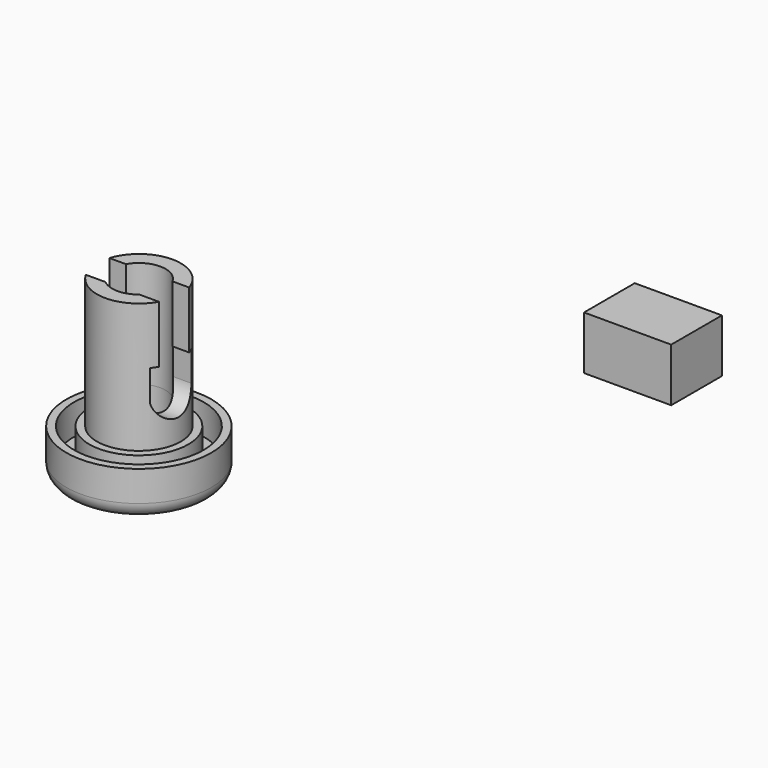
from build123d import *

# Parameters (mm, degrees)
F1_W      = 11.4284157753
F1_H      = 8.3115845919
F2_DEPTH  = 7
F4_R      = 9.5
F4_R_2    = 6.5
F4_R_3    = 5.5
F5_DEPTH  = 2
F0_R      = 5.5
F0_R_2    = 3.5
F6_DEPTH  = 7
F7_DEPTH  = 14
F8_DEPTH  = 12.5
F9_R      = 1.99999
F10_R     = 9.5
F10_R_2   = 8.5
F11_DEPTH = 4
F12_DEPTH = 4


# Not quite as in the source:
# - a fillet or chamfer is up to 0.001 mm smaller than in the source, because OpenCascade refuses the exact size


with BuildPart() as f2:
    # F1 (on Top) → F2 (new body)
    with BuildSketch(Plane.XY):
        with Locations((29.1647613049, 47.7915927768)):
            Rectangle(F1_W, F1_H)
    extrude(amount=-F2_DEPTH)


with BuildPart() as f5:
    # F4 (on face) → F5 (new body)
    with BuildSketch(Plane(origin=(0, 0, -7), x_dir=(1, 0, 0), z_dir=(0, 0, -1))):
        Circle(F4_R)
        Circle(F4_R_2, mode=Mode.SUBTRACT)
        Circle(F4_R_2)
        Circle(F4_R_3, mode=Mode.SUBTRACT)
        Circle(F4_R_3)
    extrude(amount=F5_DEPTH)

    # F0 (on Top) → F6 (join)
    with BuildSketch(Plane.XY):
        Circle(F0_R)
        Circle(F0_R_2, mode=Mode.SUBTRACT)
    extrude(amount=-F6_DEPTH)

    # F7 (add): a face of the model
    f7_faces = [f5.faces().sort_by_distance(p)[0] for p in [
        (-5.3444365081, 0, 0),
    ]]
    extrude(f7_faces, amount=F7_DEPTH)

    # F3 (on Right) → F8 (cut, symmetric)
    with BuildSketch(Plane.YZ):
        with BuildLine():
            Line((1.7, 17), (-2.7, 17))
            Line((-2.7, 17), (-2.7, 6.5))
            Line((-2.7, 6.5), (-3.5, 6.5))
            Line((-3.5, 6.5), (-3.5, 2.5))
            ThreePointArc((-3.5, 2.5), (-0.5, -0.0413812651), (2.5, 2.5))
            Line((2.5, 2.5), (2.5, 6.5))
            Line((2.5, 6.5), (1.7, 6.5))
            Line((1.7, 6.5), (1.7, 17))
        make_face()
    extrude(amount=F8_DEPTH, both=True, mode=Mode.SUBTRACT)

    # F9 (radius 2 in the source; OpenCascade refuses exactly that, so slightly less here)
    f9_edges = [f5.edges().sort_by_distance(p)[0] for p in [
        (-9.5, 0, -9),
    ]]
    fillet(f9_edges, radius=F9_R)

    # F10 (on face) → F11 (join)
    with BuildSketch(Plane(origin=(0, 0, -7), x_dir=(1, 0, 0), z_dir=(0, 0, -1))):
        Circle(F10_R)
        Circle(F10_R_2, mode=Mode.SUBTRACT)
    extrude(amount=-F11_DEPTH)


with BuildPart() as f12:
    # F4 (on face) → F12 (new body)
    with BuildSketch(Plane(origin=(0, 0, -7), x_dir=(1, 0, 0), z_dir=(0, 0, -1))):
        Circle(F4_R_2)
        Circle(F4_R_3, mode=Mode.SUBTRACT)
    extrude(amount=-F12_DEPTH)


solid = Compound([f2.part, f5.part, f12.part])
